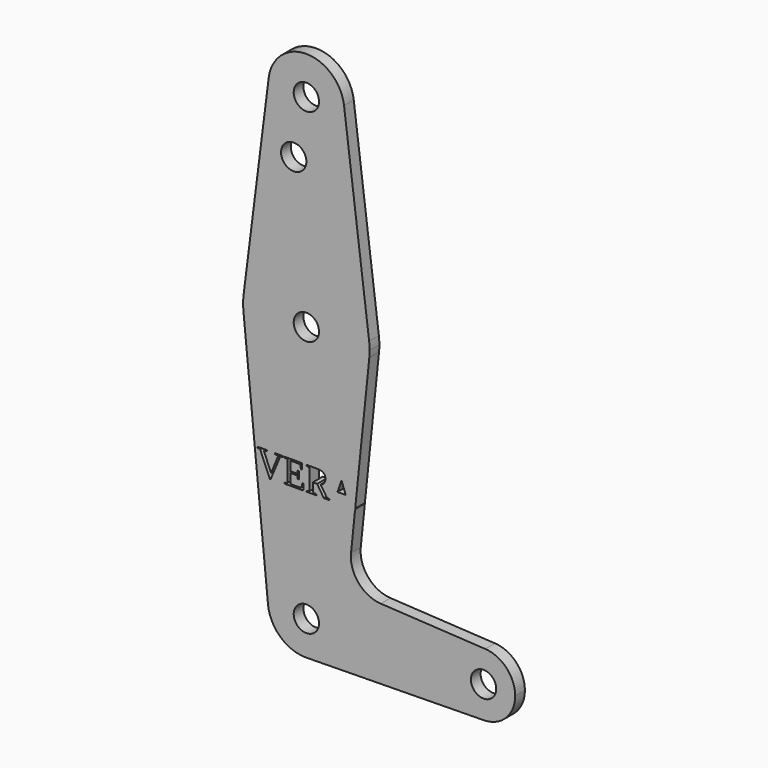
from build123d import *

# Parameters (mm, degrees)
F0_R     = 3.175
F1_DEPTH = 3.048


with BuildPart() as f1:
    # F0 (on Front) → F1 (new body)
    with BuildSketch(Plane.XZ):
        with BuildLine():
            ThreePointArc((-9.4502929642, 116.4222056828), (-0.596483242, 105.7252757886), (9.525, 115.2315806828))
            ThreePointArc((9.525, 115.2315806828), (9.5063048942, 115.8280639248), (9.4502929642, 116.4222056828))
            ThreePointArc((9.4502929642, 116.4222056828), (0, 124.7565806828), (-9.4502929642, 116.4222056828))
        make_face()
        with Locations((0, 115.2315806828)):
            Circle(F0_R, mode=Mode.SUBTRACT)
        with BuildLine():
            ThreePointArc((9.4502929642, 116.4222056828), (9.5063048942, 115.8280639248), (9.525, 115.2315806828))
            ThreePointArc((9.525, 115.2315806828), (-0.596483242, 105.7252757886), (-9.4502929642, 116.4222056828))
            Line((-9.4502929642, 116.4222056828), (-15.7504882737, 66.4159556828))
            ThreePointArc((-15.7504882737, 66.4159556828), (0, 80.3065806828), (15.7504882737, 66.4159556828))
            Line((15.7504882737, 66.4159556828), (9.4502929642, 116.4222056828))
        make_face()
        with Locations((-3.175, 100.9567806828)):
            Circle(F0_R, mode=Mode.SUBTRACT)
        with BuildLine():
            ThreePointArc((15.875, 64.4315806828), (15.8438414904, 65.4257194194), (15.7504882737, 66.4159556828))
            ThreePointArc((15.7504882737, 66.4159556828), (0, 80.3065806828), (-15.7504882737, 66.4159556828))
            ThreePointArc((-15.7504882737, 66.4159556828), (-15.8735137675, 64.6488033167), (-15.7988908218, 62.8789462115))
            ThreePointArc((-15.7988908218, 62.8789462115), (-0.0350334036, 48.5566193392), (15.7918841581, 62.8092306167))
            ThreePointArc((15.7918841581, 62.8092306167), (15.8542074228, 63.6193418048), (15.875, 64.4315806828))
        make_face()
        with Locations((0, 64.4315806828)):
            Circle(F0_R, mode=Mode.SUBTRACT)
        with BuildLine():
            ThreePointArc((15.7918841581, 62.8092306167), (-0.0350334036, 48.5566193392), (-15.7988908218, 62.8789462115))
            Line((-15.7988908218, 62.8789462115), (-9.6194684488, 0))
            ThreePointArc((-9.6194684488, 0), (-0.6064835851, 10.4451574562), (9.3848660442, 0.9315806828))
            ThreePointArc((9.3848660442, 0.9315806828), (6.6444220698, -5.7538829911), (0, -8.5923884202))
            Line((0, -8.5923884202), (44.566778303, -7.9366409191))
            ThreePointArc((44.566778303, -7.9366409191), (36.5142317093, 0.1657947093), (44.898157601, 7.9248382327))
            Line((44.898157601, 7.9248382327), (18.664461469, 9.408380228))
            ThreePointArc((18.664461469, 9.408380228), (13.0633502744, 12.1880545359), (11.2047605357, 18.158371115))
            Line((11.2047605357, 18.158371115), (12.2217881669, 28.0580733262))
            Line((12.2217881669, 28.0580733262), (9.806785479, 28.0580733262))
            Line((9.806785479, 28.0580733262), (9.806785479, 28.294084817))
            Line((9.806785479, 28.294084817), (10.6072340892, 28.4135123184))
            Line((10.6072340892, 28.4135123184), (10.0157836063, 30.1324152843))
            Line((10.0157836063, 30.1324152843), (7.6698862582, 30.1324152843))
            Line((7.6698862582, 30.1324152843), (7.0699052395, 28.4135123184))
            Line((7.0699052395, 28.4135123184), (7.8703538498, 28.294084817))
            Line((7.8703538498, 28.294084817), (7.8703538498, 28.0580733262))
            Line((7.8703538498, 28.0580733262), (5.9111741252, 28.0580733262))
            Line((5.9111741252, 28.0580733262), (5.9111741252, 28.294084817))
            Line((5.9111741252, 28.294084817), (6.5865082102, 28.4135123184))
            Line((6.5865082102, 28.4135123184), (8.6167757333, 34.0649922933))
            Line((8.6167757333, 34.0649922933), (9.4598770226, 34.0649922933))
            Line((9.4598770226, 34.0649922933), (11.5711846359, 28.4135123184))
            Line((11.5711846359, 28.4135123184), (12.2473153484, 28.3065537876))
            Line((12.2473153484, 28.3065537876), (15.7918841581, 62.8092306167))
        make_face()
        Polygon((-7.8443148705, 34.0166525904), (-5.9078832413, 34.0166525904), (-5.9078832413, 33.7806410996), (-6.5604692309, 33.6654788662), (-8.9561280379, 27.9201629973), (-9.1821872369, 27.9201629973), (-11.6034376513, 33.6654788662), (-12.2745064684, 33.7806410996), (-12.2745064684, 34.0166525904), (-9.8660518577, 34.0166525904), (-9.8660518577, 33.7806410996), (-10.666500468, 33.6654788662), (-8.862292144, 29.2793617032), (-7.0623490878, 33.6654788662), (-7.8443148705, 33.7806410996), align=None, mode=Mode.SUBTRACT)
        with BuildLine():
            Line((-5.5439137134, 28.0580733262), (-5.5439137134, 28.294084817))
            Line((-5.5439137134, 28.294084817), (-4.7790090023, 28.4135123184))
            Line((-4.7790090023, 28.4135123184), (-4.7790090023, 33.6654788662))
            Line((-4.7790090023, 33.6654788662), (-5.5439137134, 33.7806410996))
            Line((-5.5439137134, 33.7806410996), (-5.5439137134, 34.0166525904))
            Line((-5.5439137134, 34.0166525904), (-1.0739129483, 34.0166525904))
            Line((-1.0739129483, 34.0166525904), (-1.0739129483, 32.5906313539))
            Line((-1.0739129483, 32.5906313539), (-1.3667946778, 32.5906313539))
            Line((-1.3667946778, 32.5906313539), (-1.5089702747, 33.5545819006))
            add(Edge.make_bspline(
                [(-1.5089702747, 33.5545819006), (-2.0065848637, 33.6157174073), (-2.9492090708, 33.6157174073)],
                knots=[0, 0, 0, 1, 1, 1], degree=2))
            Line((-2.9492090708, 33.6157174073), (-3.9216901533, 33.6157174073))
            Line((-3.9216901533, 33.6157174073), (-3.9216901533, 31.2883028868))
            Line((-3.9216901533, 31.2883028868), (-2.3136841529, 31.2883028868))
            Line((-2.3136841529, 31.2883028868), (-2.1757738239, 31.999180871))
            Line((-2.1757738239, 31.999180871), (-1.8914226302, 31.999180871))
            Line((-1.8914226302, 31.999180871), (-1.8914226302, 30.1679591835))
            Line((-1.8914226302, 30.1679591835), (-2.1757738239, 30.1679591835))
            Line((-2.1757738239, 30.1679591835), (-2.3136841529, 30.8887894596))
            Line((-2.3136841529, 30.8887894596), (-3.9216901533, 30.8887894596))
            Line((-3.9216901533, 30.8887894596), (-3.9216901533, 28.4575867534))
            Line((-3.9216901533, 28.4575867534), (-2.7487414792, 28.4575867534))
            add(Edge.make_bspline(
                [(-2.7487414792, 28.4575867534), (-1.6028061686, 28.4575867534), (-1.2473671765, 28.5286745518)],
                knots=[0, 0, 0, 1, 1, 1], degree=2))
            Line((-1.2473671765, 28.5286745518), (-0.9942946141, 29.6305354274))
            Line((-0.9942946141, 29.6305354274), (-0.6999911286, 29.6305354274))
            Line((-0.6999911286, 29.6305354274), (-0.7852964867, 28.0580733262))
            Line((-0.7852964867, 28.0580733262), (-5.5439137134, 28.0580733262))
        make_face(mode=Mode.SUBTRACT)
        with BuildLine():
            Line((2.7065361721, 30.6712607964), (1.6359539277, 30.6712607964))
            Line((1.6359539277, 30.6712607964), (1.6359539277, 28.4135123184))
            Line((1.6359539277, 28.4135123184), (2.5373472118, 28.294084817))
            Line((2.5373472118, 28.294084817), (2.5373472118, 28.0580733262))
            Line((2.5373472118, 28.0580733262), (0.0720223624, 28.0580733262))
            Line((0.0720223624, 28.0580733262), (0.0720223624, 28.294084817))
            Line((0.0720223624, 28.294084817), (0.7786350787, 28.4135123184))
            Line((0.7786350787, 28.4135123184), (0.7786350787, 33.6654788662))
            Line((0.7786350787, 33.6654788662), (0.0137303676, 33.7806410996))
            Line((0.0137303676, 33.7806410996), (0.0137303676, 34.0166525904))
            Line((0.0137303676, 34.0166525904), (2.5871086707, 34.0166525904))
            add(Edge.make_bspline(
                [(2.5871086707, 34.0166525904), (3.7060306179, 34.0166525904), (4.2391891061, 33.6384655028)],
                knots=[0, 0, 0, 1, 1, 1], degree=2))
            add(Edge.make_bspline(
                [(4.2391891061, 33.6384655028), (4.7723475943, 33.2602784151), (4.7723475943, 32.4257076616)],
                knots=[0, 0, 0, 1, 1, 1], degree=2))
            add(Edge.make_bspline(
                [(4.7723475943, 32.4257076616), (4.7723475943, 31.8299919108), (4.4481872335, 31.3970672184)],
                knots=[0, 0, 0, 1, 1, 1], degree=2))
            add(Edge.make_bspline(
                [(4.4481872335, 31.3970672184), (4.1240268727, 30.9641425259), (3.5510592174, 30.7949535657)],
                knots=[0, 0, 0, 1, 1, 1], degree=2))
            Line((3.5510592174, 30.7949535657), (5.1633304857, 28.4135123184))
            Line((5.1633304857, 28.4135123184), (5.8073859394, 28.294084817))
            Line((5.8073859394, 28.294084817), (5.8073859394, 28.0580733262))
            Line((5.8073859394, 28.0580733262), (4.381364703, 28.0580733262))
            Line((4.381364703, 28.0580733262), (2.7065361721, 30.6712607964))
        make_face(mode=Mode.SUBTRACT)
        with BuildLine():
            ThreePointArc((9.3848660442, 0.9315806828), (-0.6064835851, 10.4451574562), (-9.6194684488, 0))
            ThreePointArc((-9.6194684488, 0), (-6.4854039547, -6.1721629528), (0, -8.5923884202))
            ThreePointArc((0, -8.5923884202), (6.6444220698, -5.7538829911), (9.3848660442, 0.9315806828))
        make_face()
        Circle(F0_R, mode=Mode.SUBTRACT)
        Polygon((12.3261370552, 28.294084817), (12.2473153484, 28.3065537876), (12.2217881669, 28.0580733262), (12.3261370552, 28.0580733262), align=None)
        Polygon((12.2217881669, 28.0580733262), (12.2473153484, 28.3065537876), (11.5711846359, 28.4135123184), (9.4598770226, 34.0649922933), (8.6167757333, 34.0649922933), (6.5865082102, 28.4135123184), (5.9111741252, 28.294084817), (5.9111741252, 28.0580733262), (7.8703538498, 28.0580733262), (7.8703538498, 28.294084817), (7.0699052395, 28.4135123184), (7.6698862582, 30.1324152843), (10.0157836063, 30.1324152843), (10.6072340892, 28.4135123184), (9.806785479, 28.294084817), (9.806785479, 28.0580733262), align=None)
        Polygon((7.8035313193, 30.5333504675), (8.8257738607, 33.4252021075), (9.8778732774, 30.5333504675), align=None, mode=Mode.SUBTRACT)
        with BuildLine():
            ThreePointArc((44.898157601, 7.9248382327), (36.5142317093, 0.1657947093), (44.566778303, -7.9366409191))
            ThreePointArc((44.566778303, -7.9366409191), (50.1037966903, -5.571219726), (52.3875, 0))
            ThreePointArc((52.3875, 0), (50.2189321892, 5.4519104584), (44.898157601, 7.9248382327))
        make_face()
        with Locations((44.45, 0)):
            Circle(F0_R, mode=Mode.SUBTRACT)
    extrude(amount=F1_DEPTH)


solid = f1.part
